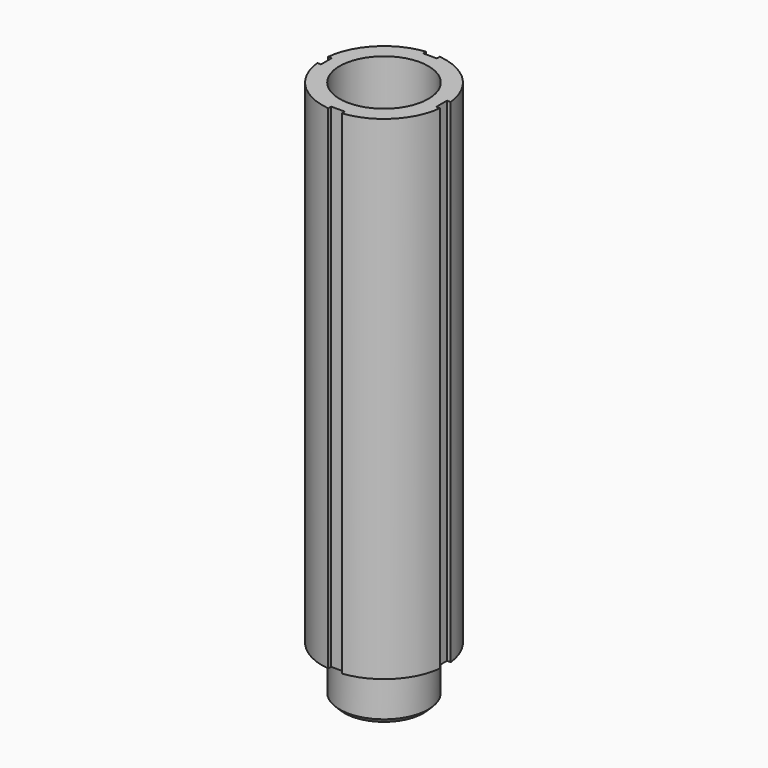
from build123d import *

# Parameters (mm, degrees)
F0_R     = 9
F1_DEPTH = 100
F2_R     = 9
F2_R_2   = 8
F3_DEPTH = 42
F4_R     = 8.975
F5_DEPTH = 10
F7_D     = 16


# Not quite as in the source:
# - a fillet or chamfer that OpenCascade refuses, or shapes differently, is made with other operations: its cross-section is extruded or revolved along the edge and cut away or added


with BuildPart() as f1:
    # F0 (on Top) → F1 (new body)
    with BuildSketch(Plane.XY):
        with BuildLine():
            Line((11.6741448398, 1.375), (12.4241448398, 1.375))
            ThreePointArc((12.4241448398, 1.375), (8.8388347648, 8.8388347648), (1.375, 12.4241448398))
            Line((1.375, 12.4241448398), (1.375, 11.6741448398))
            Line((1.375, 11.6741448398), (-1.375, 11.6741448398))
            Line((-1.375, 11.6741448398), (-1.375, 12.4241448398))
            ThreePointArc((-1.375, 12.4241448398), (-8.8388347648, 8.8388347648), (-12.4241448398, 1.375))
            Line((-12.4241448398, 1.375), (-11.6741448398, 1.375))
            Line((-11.6741448398, 1.375), (-11.6741448398, -1.375))
            Line((-11.6741448398, -1.375), (-12.4241448398, -1.375))
            ThreePointArc((-12.4241448398, -1.375), (-8.8388347648, -8.8388347648), (-1.375, -12.4241448398))
            Line((-1.375, -12.4241448398), (-1.375, -11.6741448398))
            Line((-1.375, -11.6741448398), (1.375, -11.6741448398))
            Line((1.375, -11.6741448398), (1.375, -12.4241448398))
            ThreePointArc((1.375, -12.4241448398), (8.8388347648, -8.8388347648), (12.4241448398, -1.375))
            Line((12.4241448398, -1.375), (11.6741448398, -1.375))
            Line((11.6741448398, -1.375), (11.6741448398, 1.375))
        make_face()
        Circle(F0_R, mode=Mode.SUBTRACT)
    extrude(amount=F1_DEPTH)

    # F2 (on Top) → F3 (join)
    with BuildSketch(Plane.XY):
        Circle(F2_R)
        Circle(F2_R_2, mode=Mode.SUBTRACT)
    extrude(amount=F3_DEPTH)

    # F4 (on Top) → F5 (join)
    with BuildSketch(Plane.XY):
        Circle(F4_R)
    extrude(amount=-F5_DEPTH)

    # F7 (through all)
    with Locations(Plane(origin=(0, 0, -10), x_dir=(1, 0, 0), z_dir=(0, 0, -1))):
        with Locations((0, 0)):
            Hole(F7_D / 2)

    # F8: chamfer of 1 on 1 edges, made by hand

    # F8_s1 → F8_t2 (revolve, cut)
    with BuildSketch(Plane.XZ):
        Polygon((8.975, -9), (7.975, -10), (8.975, -10), align=None)
    revolve(axis=Axis((0, 0, -10), (0, 0, 1)), mode=Mode.SUBTRACT)


solid = f1.part
